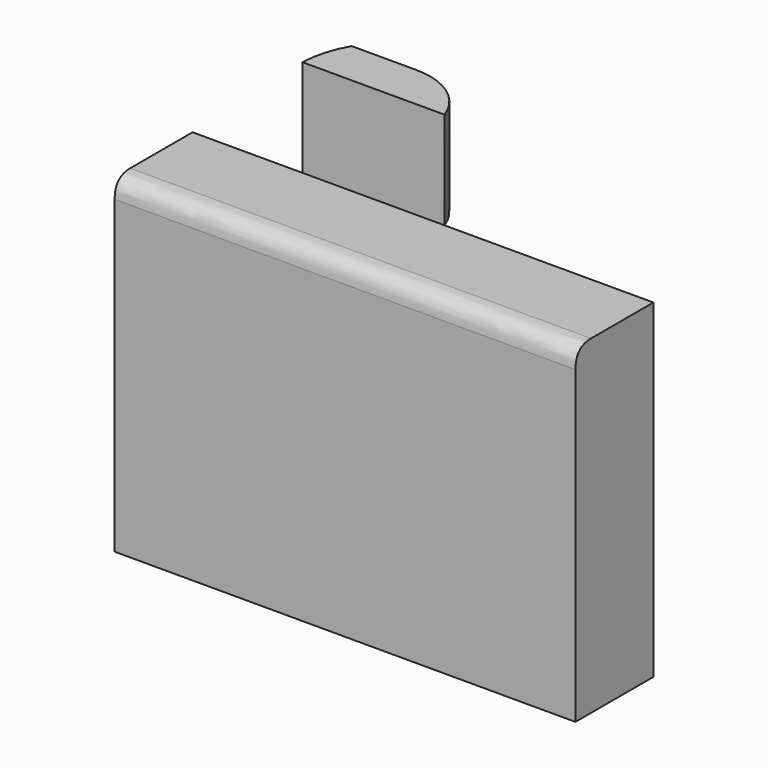
from build123d import *

# Parameters (mm, degrees)
F0_W        = 47.3044924438
F0_H        = 33.8430907577
F1_DEPTH    = 10
F3_DEPTH    = 10
F4_T1_DEPTH = 57.3044924438


# Not quite as in the source:
# - a fillet or chamfer that OpenCascade refuses, or shapes differently, is made with other operations: its cross-section is extruded or revolved along the edge and cut away or added


with BuildPart() as f1:
    # F0 (on Front) → F1 (new body)
    with BuildSketch(Plane.XZ):
        with Locations((23.6522462219, -16.9215453789)):
            Rectangle(F0_W, F0_H)
    extrude(amount=F1_DEPTH)

    # F4: fillet of radius 2 on 1 edges, made by hand

    # F4_s2 → F4_t1 (cut)
    with BuildSketch(Plane.YZ.offset(-5)):
        with BuildLine():
            add(Edge.make_bspline(
                [(-8, 0), (-10, 0), (-10, -2)],
                knots=[0, 0, 0, 1, 1, 1], degree=2, weights=[1, 1, 1]))
            Line((-10, -2), (-10, 0))
            Line((-10, 0), (-8, 0))
        make_face()
    extrude(amount=F4_T1_DEPTH, mode=Mode.SUBTRACT)


with BuildPart() as f3:
    # F2 (on face) → F3 (new body)
    with BuildSketch(Plane.XY):
        with BuildLine():
            Line((19.2758429274, 4.6487802366), (12.6155888896, 4.6487802366))
            ThreePointArc((12.6155888896, 4.6487802366), (11.6635328342, 2.4062237394), (11.2820125968, 0))
            Line((11.2820125968, 0), (25.8691551166, 0))
            ThreePointArc((25.8691551166, 0), (23.3095423248, 3.3697302602), (19.2758429274, 4.6487802366))
        make_face()
    extrude(amount=F3_DEPTH)


solid = Compound([f1.part, f3.part])
